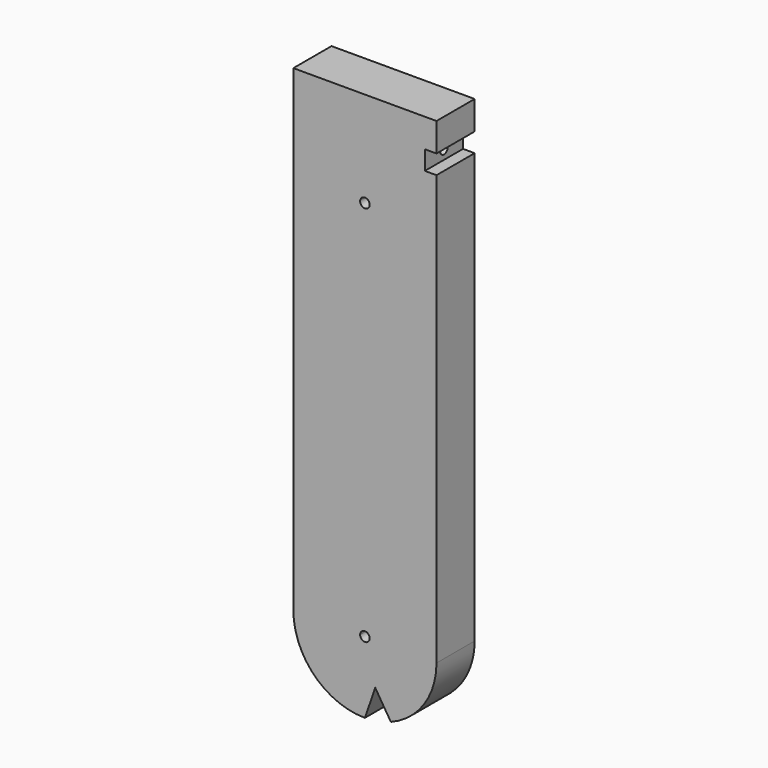
from build123d import *

# Parameters (mm, degrees)
F1_DEPTH = 3.175
F3_D     = 1.27


# Not quite as in the source:
# - a feature names something its author has since deleted; it is built from what else it names


with BuildPart() as f1:
    # F0 (on Front) → F1 (new body, symmetric)
    with BuildSketch(Plane.XZ):
        with BuildLine():
            Line((9.525, 59.69), (9.525, 63.5))
            Line((9.525, 63.5), (0, 63.5))
            Line((0, 63.5), (-9.525, 63.5))
            Line((-9.525, 63.5), (-9.525, 0))
            Line((-9.525, 0), (-0.635, 0))
            ThreePointArc((-0.635, 0), (0, 0.635), (0.635, 0))
            Line((0.635, 0), (9.525, 0))
            Line((9.525, 0), (9.525, 57.15))
            Line((9.525, 57.15), (7.9769473523, 57.15))
            Line((7.9769473523, 57.15), (7.9769473523, 59.69))
            Line((7.9769473523, 59.69), (9.525, 59.69))
        make_face()
        with BuildLine():
            ThreePointArc((0.635, 50.8), (-0.4490128061, 50.3509871939), (0, 51.435))
            ThreePointArc((0, 51.435), (0.4490128061, 51.2490128061), (0.635, 50.8))
        make_face(mode=Mode.SUBTRACT)
        with BuildLine():
            ThreePointArc((3.450873254, -8.8778994579), (7.861144724, -5.3784782818), (9.525, 0))
            Line((9.525, 0), (0.635, 0))
            ThreePointArc((0.635, 0), (0.5001354304, -0.3912665987), (0.1528281851, -0.6163347677))
            Line((0.1528281851, -0.6163347677), (1.3754536657, -5.5470129091))
            Line((1.3754536657, -5.5470129091), (3.450873254, -8.8778994579))
        make_face()
        with BuildLine():
            Line((-0.635, 0), (-9.525, 0))
            ThreePointArc((-9.525, 0), (-6.7351920908, -6.7351920908), (0, -9.525))
            Line((0, -9.525), (1.3754536657, -5.5470129091))
            Line((1.3754536657, -5.5470129091), (0.1528281851, -0.6163347677))
            ThreePointArc((0.1528281851, -0.6163347677), (-0.3912665987, -0.5001354304), (-0.635, 0))
        make_face()
    extrude(amount=F1_DEPTH, both=True)

    # F3 (through all)
    with Locations(Plane.YZ.offset(9.525)):
        with Locations((0, 58.42)):
            Hole(F3_D / 2)


solid = f1.part
